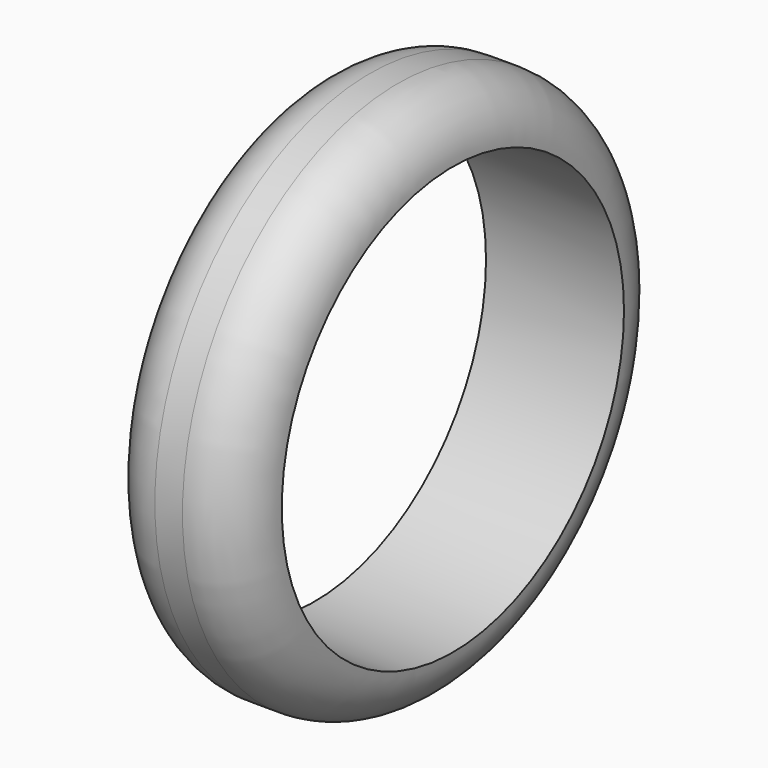
from build123d import *

# Parameters (mm, degrees)
F0_R     = 9.75
F0_R_2   = 7.75
F1_DEPTH = 5
F2_R     = 1.99999
F3_R     = 1.99999


# Not quite as in the source:
# - a fillet or chamfer is up to 0.001 mm smaller than in the source, because OpenCascade refuses the exact size


with BuildPart() as f1:
    # F0 (on Right) → F1 (new body)
    with BuildSketch(Plane.YZ):
        Circle(F0_R)
        Circle(F0_R_2, mode=Mode.SUBTRACT)
    extrude(amount=F1_DEPTH)

    # F2 (radius 2 in the source; OpenCascade refuses exactly that, so slightly less here)
    f2_edges = [f1.edges().sort_by_distance(p)[0] for p in [
        (0, -9.75, 0),
    ]]
    fillet(f2_edges, radius=F2_R)

    # F3 (radius 2 in the source; OpenCascade refuses exactly that, so slightly less here)
    f3_edges = [f1.edges().sort_by_distance(p)[0] for p in [
        (5, -9.75, 0),
    ]]
    fillet(f3_edges, radius=F3_R)


solid = f1.part
